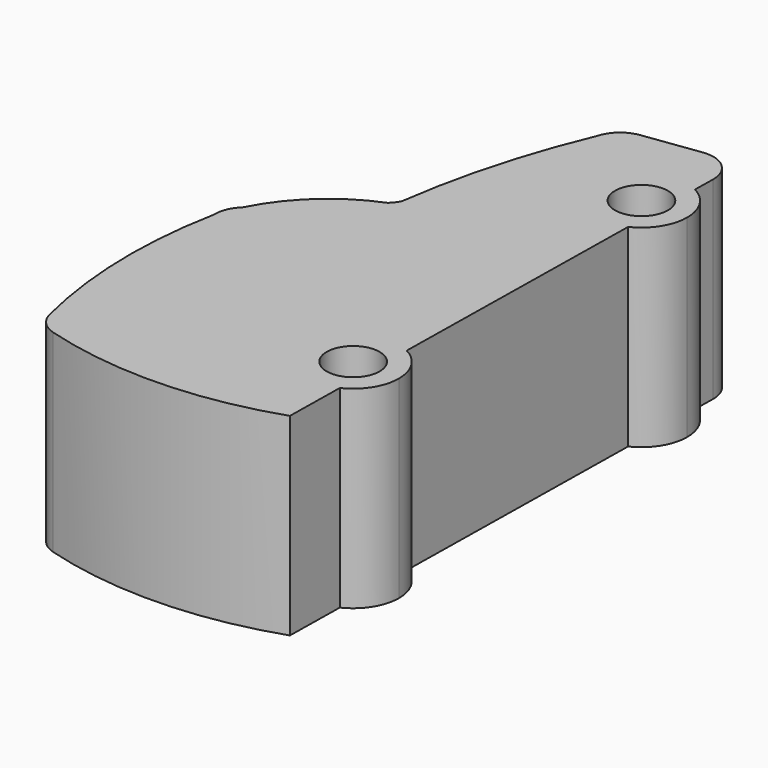
from build123d import *

# Parameters (mm, degrees)
F1_DEPTH = 19
F2_R     = 7.5
F2_R_2   = 2.5
F3_DEPTH = 5


# Not quite as in the source:
# - a feature names something its author has since deleted; it is built from what else it names


with BuildPart() as f1:
    # F0 (on Top) → F1 (new body)
    with BuildSketch(Plane.XY):
        with BuildLine():
            Line((-18.4867138529, 55.6857541377), (-24.0573941449, 54.93137017))
            ThreePointArc((-24.0573941449, 54.93137017), (-25.6311486072, 54.2155115142), (-26.5485038183, 52.7500367996))
            ThreePointArc((-26.5485038183, 52.7500367996), (-29.5944451056, 44.0185448748), (-31.46174181, 34.9615082415))
            ThreePointArc((-31.46174181, 34.9615082415), (-31.7590054988, 34.4640245193), (-32.1463756641, 34.032979151))
            ThreePointArc((-32.1463756641, 34.032979151), (-36.9518125946, 31.0156700781), (-40.3745702721, 26.4900642606))
            ThreePointArc((-40.3745702721, 26.4900642606), (-41.1187881848, 25.4271596859), (-41.3445519166, 24.1494049466))
            ThreePointArc((-41.3445519166, 24.1494049466), (-42.2235056982, 13.7140274197), (-40.8158360427, 3.3367382737))
            ThreePointArc((-40.8158360427, 3.3367382737), (-40.0672712074, 1.9827956506), (-38.7436286277, 1.181871022))
            ThreePointArc((-38.7436286277, 1.181871022), (-27.2787715313, -0.3216500473), (-15.8934134801, 1.6975443206))
            Line((-15.8934134801, 1.6975443206), (-15.7980047108, 7.7090638021))
            ThreePointArc((-15.7980047108, 7.7090638021), (-22.2332162759, 11.8428335239), (-15.670064806, 15.7703063478))
            Line((-15.670064806, 15.7703063478), (-15.2468750991, 42.4346600078))
            ThreePointArc((-15.2468750991, 42.4346600078), (-21.6820866642, 46.5684297296), (-15.1189351942, 50.4959025535))
            Line((-15.1189351942, 50.4959025535), (-15.0845049847, 52.6652825485))
            ThreePointArc((-15.0845049847, 52.6652825485), (-16.0924041894, 54.9563331626), (-18.4867138529, 55.6857541377))
        make_face()
        with BuildLine():
            ThreePointArc((-12.6826533059, 46.4970192649), (-13.3396901586, 48.8383082793), (-15.1189351942, 50.4959025535))
            Line((-15.1189351942, 50.4959025535), (-15.1565415969, 48.1263968586))
            ThreePointArc((-15.1565415969, 48.1263968586), (-14.7303186587, 47.3607638906), (-14.5826533059, 46.4970192649))
            ThreePointArc((-14.5826533059, 46.4970192649), (-14.7443342143, 45.5944673231), (-15.2092686964, 44.8041657027))
            Line((-15.2092686964, 44.8041657027), (-15.2468750991, 42.4346600078))
            ThreePointArc((-15.2468750991, 42.4346600078), (-13.377327963, 44.0950411146), (-12.6826533059, 46.4970192649))
        make_face()
        with BuildLine():
            Line((-15.1565415969, 48.1263968586), (-15.1189351942, 50.4959025535))
            ThreePointArc((-15.1189351942, 50.4959025535), (-21.6820866642, 46.5684297296), (-15.2468750991, 42.4346600078))
            Line((-15.2468750991, 42.4346600078), (-15.2092686964, 44.8041657027))
            ThreePointArc((-15.2092686964, 44.8041657027), (-19.7823259129, 46.5382786445), (-15.1565415969, 48.1263968586))
        make_face()
        with BuildLine():
            Line((-15.7076712086, 13.4008006529), (-15.670064806, 15.7703063478))
            ThreePointArc((-15.670064806, 15.7703063478), (-22.2332162759, 11.8428335239), (-15.7980047108, 7.7090638021))
            Line((-15.7980047108, 7.7090638021), (-15.7603983081, 10.0785694971))
            ThreePointArc((-15.7603983081, 10.0785694971), (-20.3334555246, 11.8126824388), (-15.7076712086, 13.4008006529))
        make_face()
        with BuildLine():
            ThreePointArc((-13.2337829176, 11.7714230593), (-13.8908197703, 14.1127120736), (-15.670064806, 15.7703063478))
            Line((-15.670064806, 15.7703063478), (-15.7076712086, 13.4008006529))
            ThreePointArc((-15.7076712086, 13.4008006529), (-15.3007413769, 12.6881066805), (-15.1362247549, 11.8840800221))
            Line((-15.1362247549, 11.8840800221), (-15.1362247549, 11.6587660965))
            ThreePointArc((-15.1362247549, 11.6587660965), (-15.3155945916, 10.8162449502), (-15.7603983081, 10.0785694971))
            Line((-15.7603983081, 10.0785694971), (-15.7980047108, 7.7090638021))
            ThreePointArc((-15.7980047108, 7.7090638021), (-13.9284575747, 9.3694449089), (-13.2337829176, 11.7714230593))
        make_face()
    extrude(amount=F1_DEPTH)


with BuildPart() as f3:
    # F2 (on Top) → F3 (new body)
    with BuildSketch(Plane.XY):
        with Locations((-42.5560415272, 22.8924162194)):
            Circle(F2_R)
        with BuildLine():
            ThreePointArc((-36.829554944, 26.4032928604), (-36.4020595038, 25.5845173749), (-36.0909286598, 24.7148374079))
            ThreePointArc((-36.0909286598, 24.7148374079), (-35.9865291403, 24.2925627739), (-35.9096801821, 23.8644163459))
            ThreePointArc((-35.9096801821, 23.8644163459), (-35.8566790413, 23.3797001801), (-35.8389809069, 22.8924162194))
            ThreePointArc((-35.8389809069, 22.8924162194), (-35.9042334364, 21.9584180933), (-36.0987232404, 21.0425665179))
            ThreePointArc((-36.0987232404, 21.0425665179), (-36.3395382025, 20.3480125978), (-36.6548093118, 19.6839334447))
            ThreePointArc((-36.6548093118, 19.6839334447), (-36.992942718, 19.1279992639), (-37.3832803945, 18.6073904739))
            ThreePointArc((-37.3832803945, 18.6073904739), (-37.7906796134, 18.1584718591), (-38.2368936112, 17.7481121212))
            ThreePointArc((-38.2368936112, 17.7481121212), (-38.7721055408, 17.3425755167), (-39.3451335754, 16.9925032116))
            ThreePointArc((-39.3451335754, 16.9925032116), (-39.6838378223, 16.8204026117), (-40.0317304914, 16.6677268962))
            ThreePointArc((-40.0317304914, 16.6677268962), (-40.9887550369, 16.3607612658), (-41.9808680572, 16.2000265973))
            ThreePointArc((-41.9808680572, 16.2000265973), (-42.4514489154, 16.1761699642), (-42.9225444398, 16.1853617996))
            ThreePointArc((-42.9225444398, 16.1853617996), (-43.9153904074, 16.3143409692), (-44.8780365625, 16.589461164))
            ThreePointArc((-44.8780365625, 16.589461164), (-45.435948651, 16.8240524916), (-45.9704801387, 17.1079099879))
            ThreePointArc((-45.9704801387, 17.1079099879), (-46.5079882683, 17.4609320456), (-47.0092746326, 17.8637366429))
            ThreePointArc((-47.0092746326, 17.8637366429), (-47.2892940825, 18.1263671615), (-47.5538518611, 18.4045664847))
            ThreePointArc((-47.5538518611, 18.4045664847), (-48.116773764, 19.1245042824), (-48.5767615095, 19.9141895206))
            ThreePointArc((-48.5767615095, 19.9141895206), (-48.7708001482, 20.3437540886), (-48.9342357685, 20.7858689034))
            ThreePointArc((-48.9342357685, 20.7858689034), (-49.2009974057, 21.910853818), (-49.2708867143, 23.0649198099))
            ThreePointArc((-49.2708867143, 23.0649198099), (-49.2522737571, 23.4209777562), (-49.2147939886, 23.7755464664))
            ThreePointArc((-49.2147939886, 23.7755464664), (-49.043482284, 24.6336846657), (-48.7620670518, 25.4622704105))
            ThreePointArc((-48.7620670518, 25.4622704105), (-48.630264893, 25.7599437045), (-48.4841948015, 26.0508813738))
            ThreePointArc((-48.4841948015, 26.0508813738), (-47.8022969745, 27.0871399477), (-46.9414713871, 27.9803340961))
            ThreePointArc((-46.9414713871, 27.9803340961), (-46.6471161076, 28.2198933102), (-46.3397008388, 28.4424455517))
            ThreePointArc((-46.3397008388, 28.4424455517), (-45.76910866, 28.7911536246), (-45.1666718224, 29.0813994023))
            ThreePointArc((-45.1666718224, 29.0813994023), (-44.8430367604, 29.2081549869), (-44.5132782297, 29.3180000735))
            ThreePointArc((-44.5132782297, 29.3180000735), (-43.5454522375, 29.536208045), (-42.5560415272, 29.6094768397))
            ThreePointArc((-42.5560415272, 29.6094768397), (-42.231677867, 29.6016405853), (-41.9080710248, 29.5781501061))
            ThreePointArc((-41.9080710248, 29.5781501061), (-40.8244371879, 29.3824431676), (-39.7873399477, 29.012317766))
            ThreePointArc((-39.7873399477, 29.012317766), (-39.5219662451, 28.8851860764), (-39.2624151007, 28.7465539304))
            ThreePointArc((-39.2624151007, 28.7465539304), (-38.1965318152, 28.0025608795), (-37.2939053957, 27.0672008498))
            ThreePointArc((-37.2939053957, 27.0672008498), (-37.0517113458, 26.7422542199), (-36.829554944, 26.4032928604))
        make_face(mode=Mode.SUBTRACT)
        with BuildLine():
            Line((-36.0987232404, 21.0425665179), (-39.1638805296, 22.0303003532))
            ThreePointArc((-39.1638805296, 22.0303003532), (-39.2648640734, 21.7015547799), (-39.3976232849, 21.3843067384))
            Line((-39.3976232849, 21.3843067384), (-36.6548093118, 19.6839334447))
            ThreePointArc((-36.6548093118, 19.6839334447), (-36.3395382025, 20.3480125978), (-36.0987232404, 21.0425665179))
        make_face()
        with BuildLine():
            ThreePointArc((-39.132827379, 23.6215286224), (-39.0752909243, 23.2589885054), (-39.0560415272, 22.8924162194))
            ThreePointArc((-39.0560415272, 22.8924162194), (-39.0569583824, 22.8123091265), (-39.0597084679, 22.732244003))
            Line((-39.0597084679, 22.732244003), (-35.9096801821, 23.8644163459))
            ThreePointArc((-35.9096801821, 23.8644163459), (-35.9865291403, 24.2925627739), (-36.0909286598, 24.7148374079))
            Line((-36.0909286598, 24.7148374079), (-39.132827379, 23.6215286224))
        make_face()
        with BuildLine():
            ThreePointArc((-39.8927436716, 25.163284893), (-39.6476626206, 24.8395505589), (-39.4417244656, 24.4896103968))
            Line((-39.4417244656, 24.4896103968), (-36.829554944, 26.4032928604))
            ThreePointArc((-36.829554944, 26.4032928604), (-37.0517113458, 26.7422542199), (-37.2939053957, 27.0672008498))
            Line((-37.2939053957, 27.0672008498), (-39.8927436716, 25.163284893))
        make_face()
        with BuildLine():
            ThreePointArc((-39.0597084679, 22.732244003), (-39.0569583824, 22.8123091265), (-39.0560415272, 22.8924162194))
            ThreePointArc((-39.0560415272, 22.8924162194), (-39.0752909243, 23.2589885054), (-39.132827379, 23.6215286224))
            ThreePointArc((-39.132827379, 23.6215286224), (-39.2585849208, 24.0657788782), (-39.4417244656, 24.4896103968))
            ThreePointArc((-39.4417244656, 24.4896103968), (-39.6476626206, 24.8395505589), (-39.8927436716, 25.163284893))
            ThreePointArc((-39.8927436716, 25.163284893), (-40.1868435925, 25.4686346004), (-40.515704619, 25.7361857779))
            ThreePointArc((-40.515704619, 25.7361857779), (-40.763863783, 25.8987593358), (-41.024899288, 26.0397330836))
            ThreePointArc((-41.024899288, 26.0397330836), (-41.4567348008, 26.2152952003), (-41.9080710248, 26.3319124366))
            ThreePointArc((-41.9080710248, 26.3319124366), (-42.2306469668, 26.3772574468), (-42.5560415272, 26.3924162194))
            ThreePointArc((-42.5560415272, 26.3924162194), (-42.8814360875, 26.3772574468), (-43.2040120295, 26.3319124366))
            ThreePointArc((-43.2040120295, 26.3319124366), (-43.5508479772, 26.2480622268), (-43.8873439447, 26.1293335606))
            ThreePointArc((-43.8873439447, 26.1293335606), (-44.2536485399, 25.9531563963), (-44.5970572739, 25.7356986046))
            ThreePointArc((-44.5970572739, 25.7356986046), (-44.8959140549, 25.4952985745), (-45.1666718224, 25.2236411038))
            ThreePointArc((-45.1666718224, 25.2236411038), (-45.3353778089, 25.0196890822), (-45.4881886835, 24.8035711199))
            ThreePointArc((-45.4881886835, 24.8035711199), (-45.6536452917, 24.5217875454), (-45.7921014478, 24.2258014563))
            ThreePointArc((-45.7921014478, 24.2258014563), (-45.9031313374, 23.9156414157), (-45.9845082279, 23.5964162775))
            ThreePointArc((-45.9845082279, 23.5964162775), (-46.0424319056, 23.2007701216), (-46.0548500683, 22.8010992291))
            ThreePointArc((-46.0548500683, 22.8010992291), (-46.0230139848, 22.4127267598), (-45.9482025247, 22.0303003532))
            ThreePointArc((-45.9482025247, 22.0303003532), (-45.8472189809, 21.7015547799), (-45.7144597694, 21.3843067384))
            ThreePointArc((-45.7144597694, 21.3843067384), (-45.5661116717, 21.1065053244), (-45.3933928705, 20.8431633424))
            ThreePointArc((-45.3933928705, 20.8431633424), (-45.1504482326, 20.543149558), (-44.875940706, 20.2717163511))
            ThreePointArc((-44.875940706, 20.2717163511), (-44.5866141985, 20.0416663836), (-44.2746392941, 19.8434128224))
            ThreePointArc((-44.2746392941, 19.8434128224), (-43.7117052617, 19.5887150628), (-43.112755495, 19.4369756458))
            ThreePointArc((-43.112755495, 19.4369756458), (-43.0178235038, 19.4230131864), (-42.9225444398, 19.4116583113))
            ThreePointArc((-42.9225444398, 19.4116583113), (-42.4507482802, 19.3940003877), (-41.9808680572, 19.4400003292))
            ThreePointArc((-41.9808680572, 19.4400003292), (-41.6889373989, 19.501526892), (-41.4033071565, 19.5876918027))
            ThreePointArc((-41.4033071565, 19.5876918027), (-41.0515300083, 19.7322825056), (-40.7175188239, 19.9141895206))
            ThreePointArc((-40.7175188239, 19.9141895206), (-40.4204666328, 20.1194539279), (-40.1461427954, 20.3542302328))
            ThreePointArc((-40.1461427954, 20.3542302328), (-39.9626809244, 20.5419948138), (-39.7938083043, 20.742981963))
            ThreePointArc((-39.7938083043, 20.742981963), (-39.5783993711, 21.0529469508), (-39.3976232849, 21.3843067384))
            ThreePointArc((-39.3976232849, 21.3843067384), (-39.2648640734, 21.7015547799), (-39.1638805296, 22.0303003532))
            ThreePointArc((-39.1638805296, 22.0303003532), (-39.0939585105, 22.3786252254), (-39.0597084679, 22.732244003))
        make_face()
        with Locations((-42.5560415272, 22.8924162194)):
            Circle(F2_R_2, mode=Mode.SUBTRACT)
        with BuildLine():
            ThreePointArc((-41.024899288, 26.0397330836), (-40.763863783, 25.8987593358), (-40.515704619, 25.7361857779))
            Line((-40.515704619, 25.7361857779), (-39.2624151007, 28.7465539304))
            ThreePointArc((-39.2624151007, 28.7465539304), (-39.5219662451, 28.8851860764), (-39.7873399477, 29.012317766))
            Line((-39.7873399477, 29.012317766), (-41.024899288, 26.0397330836))
        make_face()
        with BuildLine():
            ThreePointArc((-43.8873439447, 26.1293335606), (-43.5508479772, 26.2480622268), (-43.2040120295, 26.3319124366))
            Line((-43.2040120295, 26.3319124366), (-44.5132782297, 29.3180000735))
            ThreePointArc((-44.5132782297, 29.3180000735), (-44.8430367604, 29.2081549869), (-45.1666718224, 29.0813994023))
            Line((-45.1666718224, 29.0813994023), (-43.8873439447, 26.1293335606))
        make_face()
        with BuildLine():
            ThreePointArc((-45.1666718224, 25.2236411038), (-44.8959140549, 25.4952985745), (-44.5970572739, 25.7356986046))
            Line((-44.5970572739, 25.7356986046), (-46.3397008388, 28.4424455517))
            ThreePointArc((-46.3397008388, 28.4424455517), (-46.6471161076, 28.2198933102), (-46.9414713871, 27.9803340961))
            Line((-46.9414713871, 27.9803340961), (-45.1666718224, 25.2236411038))
        make_face()
        with BuildLine():
            ThreePointArc((-46.0548500683, 22.8010992291), (-46.0424319056, 23.2007701216), (-45.9845082279, 23.5964162775))
            Line((-45.9845082279, 23.5964162775), (-49.2147939886, 23.7755464664))
            ThreePointArc((-49.2147939886, 23.7755464664), (-49.2522737571, 23.4209777562), (-49.2708867143, 23.0649198099))
            Line((-49.2708867143, 23.0649198099), (-46.0548500683, 22.8010992291))
        make_face()
        with BuildLine():
            Line((-48.5767615095, 19.9141895206), (-45.7144597694, 21.3843067384))
            ThreePointArc((-45.7144597694, 21.3843067384), (-45.8472189809, 21.7015547799), (-45.9482025247, 22.0303003532))
            Line((-45.9482025247, 22.0303003532), (-48.9342357685, 20.7858689034))
            ThreePointArc((-48.9342357685, 20.7858689034), (-48.7708001482, 20.3437540886), (-48.5767615095, 19.9141895206))
        make_face()
        with BuildLine():
            Line((-47.0092746326, 17.8637366429), (-44.875940706, 20.2717163511))
            ThreePointArc((-44.875940706, 20.2717163511), (-45.1504482326, 20.543149558), (-45.3933928705, 20.8431633424))
            Line((-45.3933928705, 20.8431633424), (-47.5538518611, 18.4045664847))
            ThreePointArc((-47.5538518611, 18.4045664847), (-47.2892940825, 18.1263671615), (-47.0092746326, 17.8637366429))
        make_face()
        with BuildLine():
            Line((-44.8780365625, 16.589461164), (-43.112755495, 19.4369756458))
            ThreePointArc((-43.112755495, 19.4369756458), (-43.7117052617, 19.5887150628), (-44.2746392941, 19.8434128224))
            Line((-44.2746392941, 19.8434128224), (-45.9704801387, 17.1079099879))
            ThreePointArc((-45.9704801387, 17.1079099879), (-45.435948651, 16.8240524916), (-44.8780365625, 16.589461164))
        make_face()
        with BuildLine():
            ThreePointArc((-42.5560415272, 26.3924162194), (-42.2306469668, 26.3772574468), (-41.9080710248, 26.3319124366))
            Line((-41.9080710248, 26.3319124366), (-41.9080710248, 29.5781501061))
            ThreePointArc((-41.9080710248, 29.5781501061), (-42.231677867, 29.6016405853), (-42.5560415272, 29.6094768397))
            Line((-42.5560415272, 29.6094768397), (-42.5560415272, 26.3924162194))
        make_face()
        with BuildLine():
            Line((-41.9808680572, 16.2000265973), (-41.9808680572, 19.4400003292))
            ThreePointArc((-41.9808680572, 19.4400003292), (-42.4507482802, 19.3940003877), (-42.9225444398, 19.4116583113))
            Line((-42.9225444398, 19.4116583113), (-42.9225444398, 16.1853617996))
            ThreePointArc((-42.9225444398, 16.1853617996), (-42.4514489154, 16.1761699642), (-41.9808680572, 16.2000265973))
        make_face()
        with BuildLine():
            Line((-39.3451335754, 16.9925032116), (-40.7175188239, 19.9141895206))
            ThreePointArc((-40.7175188239, 19.9141895206), (-41.0515300083, 19.7322825056), (-41.4033071565, 19.5876918027))
            Line((-41.4033071565, 19.5876918027), (-40.0317304914, 16.6677268962))
            ThreePointArc((-40.0317304914, 16.6677268962), (-39.6838378223, 16.8204026117), (-39.3451335754, 16.9925032116))
        make_face()
        with BuildLine():
            Line((-37.3832803945, 18.6073904739), (-39.7938083043, 20.742981963))
            ThreePointArc((-39.7938083043, 20.742981963), (-39.9626809244, 20.5419948138), (-40.1461427954, 20.3542302328))
            Line((-40.1461427954, 20.3542302328), (-38.2368936112, 17.7481121212))
            ThreePointArc((-38.2368936112, 17.7481121212), (-37.7906796134, 18.1584718591), (-37.3832803945, 18.6073904739))
        make_face()
        with BuildLine():
            ThreePointArc((-45.7921014478, 24.2258014563), (-45.6536452917, 24.5217875454), (-45.4881886835, 24.8035711199))
            Line((-45.4881886835, 24.8035711199), (-48.4841948015, 26.0508813738))
            ThreePointArc((-48.4841948015, 26.0508813738), (-48.630264893, 25.7599437045), (-48.7620670518, 25.4622704105))
            Line((-48.7620670518, 25.4622704105), (-45.7921014478, 24.2258014563))
        make_face()
    extrude(amount=-F3_DEPTH)


solid = Compound([f1.part, f3.part])
